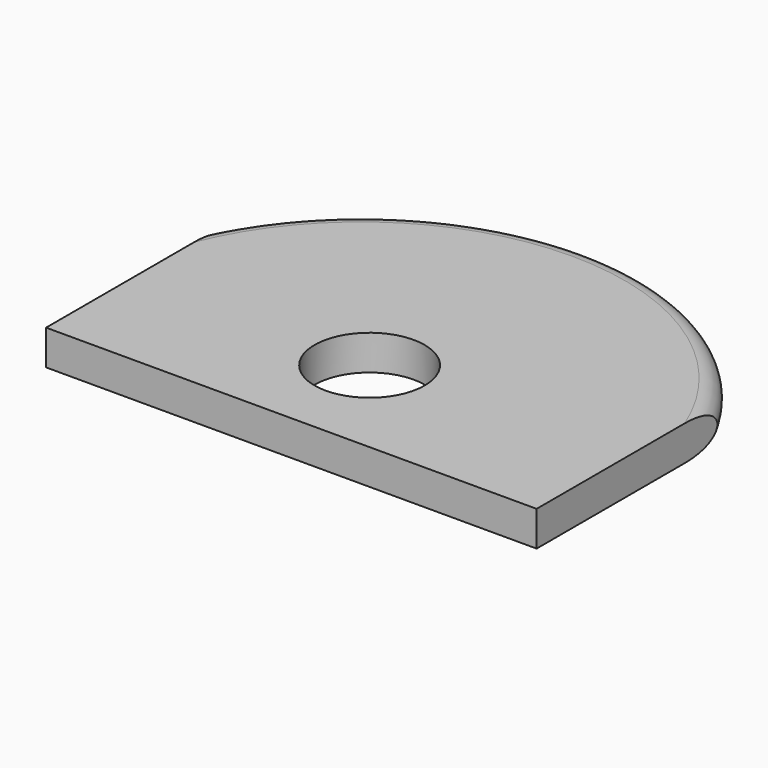
from build123d import *

# Parameters (mm, degrees)
F0_R        = 15.7049958866
F1_DEPTH    = 10
F2_R        = 5.08
F3_T2_ANGLE = 138.8894896051


# Not quite as in the source:
# - a fillet or chamfer that OpenCascade refuses, or shapes differently, is made with other operations: its cross-section is extruded or revolved along the edge and cut away or added


with BuildPart() as f1:
    # F0 (on Top) → F1 (new body)
    with BuildSketch(Plane.XY):
        with BuildLine():
            Line((-67.6743760705, 33.6404591799), (-67.6743760705, -30.8862738311))
            Line((-67.6743760705, -30.8862738311), (72.3958462477, -30.8862738311))
            Line((72.3958462477, -30.8862738311), (72.3958462477, 33.6404591799))
            ThreePointArc((72.3958462477, 33.6404591799), (2.3607350886, 74.4084313611), (-67.6743760705, 33.6404591799))
        make_face()
        Circle(F0_R, mode=Mode.SUBTRACT)
    extrude(amount=F1_DEPTH)

    # F2
    f2_edges = [f1.edges().sort_by_distance(p)[0] for p in [
        (2.360735, 74.408431, 10),
    ]]
    fillet(f2_edges, radius=F2_R)

    # F3: fillet of radius 5.08 on 1 edges, made by hand

    # F3_s1 → F3_t2 (revolve, cut)
    with BuildSketch(Plane(origin=(2.3069814419, -6.152208534, 0), x_dir=(0, 0, 1), z_dir=(0.351110531, -0.9363340189, 0))):
        with BuildLine():
            ThreePointArc((4.92, -80.5978917459), (1.4317675513, -79.0554933848), (0, -75.5204120561))
            Line((0, -75.5204120561), (0, -80.5978917459))
            Line((0, -80.5978917459), (4.92, -80.5978917459))
        make_face()
    revolve(axis=Axis((2.3607350886, -6.1320517619, 0), (0, 0, 1)), revolution_arc=F3_T2_ANGLE, mode=Mode.SUBTRACT)


solid = f1.part
